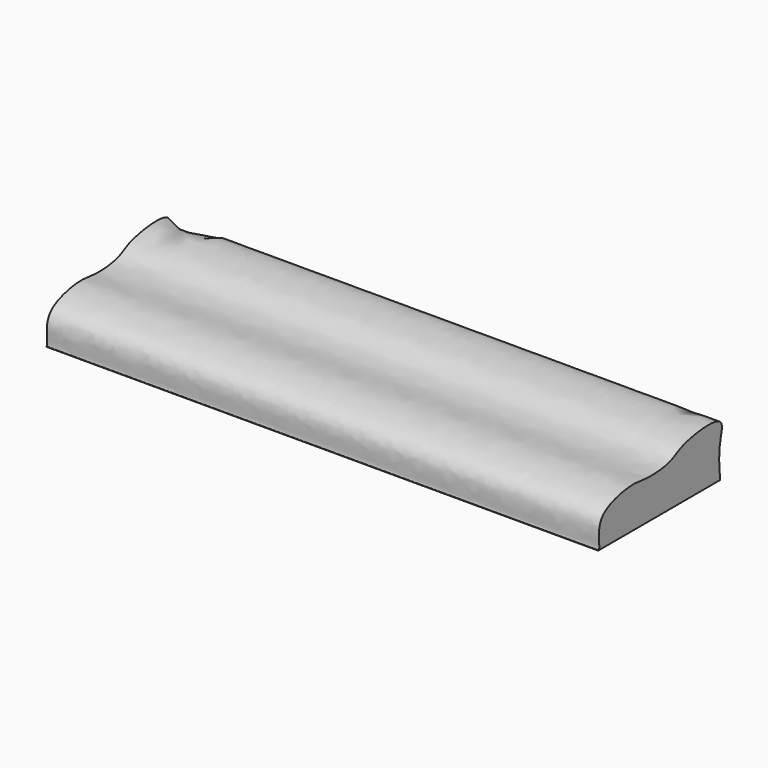
from build123d import *

# Parameters (mm, degrees)
F1_DEPTH = 100


with BuildPart() as f1:
    # F0 (on Right) → F1 (new body)
    with BuildSketch(Plane.YZ):
        with BuildLine():
            Line((-27.4707945164, -0.0370952116), (0, 0))
            add(Edge.make_bspline(
                [(0, 0), (-0.1723960733, 2.0201415213), (-0.4756077019, 5.5731830097), (1.6875698156, 10.6917174648), (-8.8251839298, 9.3987754232), (-10.8082568794, 7.2964584479), (-16.6368751127, 6.801009759), (-19.5154827985, 7.6906763858), (-26.6291772402, 6.295671632), (-27.6710413001, 2.8451492855), (-27.2041217809, 0.1175378731), (-27.4491996919, -0.0307887023), (-27.4707945164, -0.0370952116)],
                knots=[0, 0, 0, 0, 0.1239812913, 0.2180593128, 0.3637810943, 0.4581840847, 0.573759625, 0.6680006292, 0.7976881814, 0.8920911723, 0.9728419475, 0.9797844728, 0.9797844728, 0.9797844728, 0.9797844728], degree=3))
        make_face()
    extrude(amount=F1_DEPTH)


with BuildPart() as f1b:
    # F0 (on Right) → F1, piece 2 (new body)
    with BuildSketch(Plane.YZ):
        with BuildLine():
            add(Edge.make_bspline(
                [(-27.4707945164, -0.0370952116), (-27.5003464308, -0.0457254936), (-27.5340041528, -0.0441752313), (-27.5698380839, -0.0372289552)],
                knots=[0.9797844728, 0.9797844728, 0.9797844728, 0.9797844728, 0.9892851247, 0.9892851247, 0.9892851247, 0.9892851247], degree=3))
            Line((-27.4707945164, -0.0370952116), (-27.5698380839, -0.0372289552))
        make_face()
    extrude(amount=F1_DEPTH)


solid = Compound([f1.part, f1b.part])
